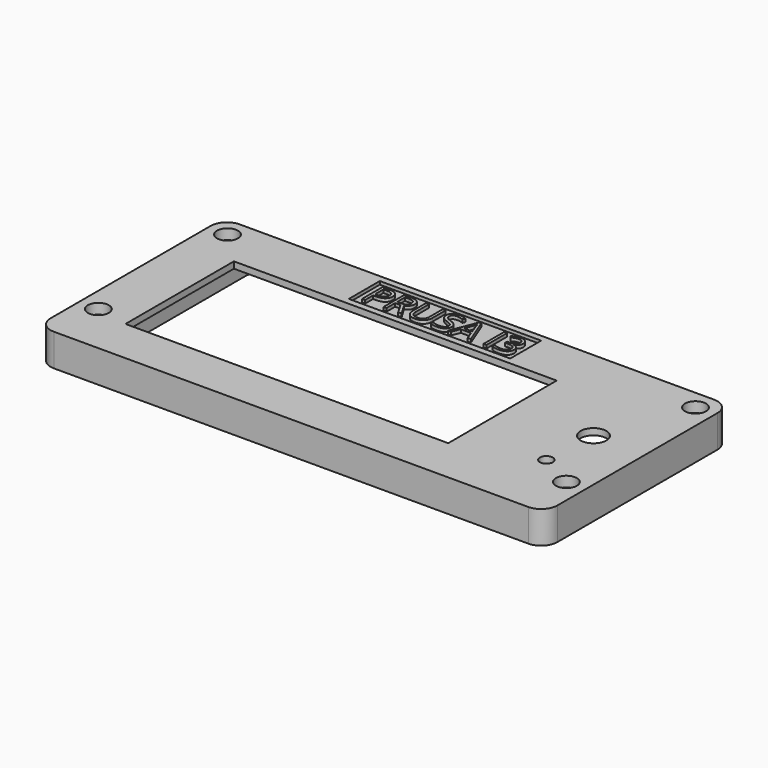
from build123d import *

# Parameters (mm, degrees)
F0_W           = 157
F0_H           = 72
F1_DEPTH       = 10
F2_W           = 100
F2_H           = 42
F2_R           = 4
F3_DEPTH       = 10.001
F4_R           = 4
F4_W           = 100
F4_H           = 42
F5_DEPTH       = 8
F6_R           = 5
F8_D           = 3.3
F8_DEPTH       = 12
F8_CBORE_D     = 6.5
F8_CBORE_DEPTH = 3.2
F8_TIP         = 0.9914200214
F9_W           = 50
F9_H           = 12
F10_DEPTH      = 1
F11_TEXT_SIZE  = 11.1111111111
F12_DEPTH      = 1
F13_R          = 2
F15_D          = 4


# Not quite as in the source:
# - Text() gives the source's letters only with a copy of the font that has no kerning and outlines rounded to 1/6400 em; it was checked with that copy


with BuildPart() as f1:
    # F0 (on Top) → F1 (new body)
    with BuildSketch(Plane.XY):
        with Locations((3.5, 8.5)):
            Rectangle(F0_W, F0_H)
    extrude(amount=F1_DEPTH)

    # F2 (on face) → F3 (cut, through all)
    with BuildSketch(Plane.XY.offset(10)):
        with Locations((-9, 7.5)):
            Rectangle(F2_W, F2_H)
        with Locations((66, 11.5)):
            Circle(F2_R)
    extrude(amount=-F3_DEPTH, mode=Mode.SUBTRACT)

    # F4 (on face) → F5 (cut)
    with BuildSketch(Plane(origin=(0, 0, 0), x_dir=(1, 0, 0), z_dir=(0, 0, -1))):
        with BuildLine():
            Line((71, 25.5), (-64, 25.5))
            Line((-64, 25.5), (-64, -41.5))
            Line((-64, -41.5), (70.8038475773, -41.5))
            ThreePointArc((70.8038475773, -41.5), (71.3859855926, -34.6645246646), (78, -32.8431457505))
            Line((78, -32.8431457505), (78, 5.5))
            Line((78, 5.5), (71, 5.5))
            Line((71, 5.5), (71, 25.5))
        make_face()
        with Locations((66, -11.5)):
            Circle(F4_R, mode=Mode.SUBTRACT)
        with Locations((-9, -7.5)):
            Rectangle(F4_W, F4_H, mode=Mode.SUBTRACT)
    extrude(amount=-F5_DEPTH, mode=Mode.SUBTRACT)

    # F6
    f6_edges = [f1.edges().sort_by_distance(p)[0] for p in [
        (-75, -27.5, 5),
        (-75, 44.5, 5),
        (82, 44.5, 5),
        (82, -27.5, 5),
    ]]
    fillet(f6_edges, radius=F6_R)

    # F8
    with Locations(Plane.XY.offset(10)):
        with Locations((-69, 38.5), (-69, -11.5), (76, 38.5), (76, -11.5)):
            CounterBoreHole(F8_D / 2, F8_CBORE_D / 2, F8_CBORE_DEPTH, depth=F8_DEPTH)
            with Locations((0, 0, -(F8_DEPTH + F8_TIP / 2))):  # 118° drill point
                Cone(0, F8_D / 2, F8_TIP, mode=Mode.SUBTRACT)

    # F9 (on face) → F10 (cut)
    with BuildSketch(Plane.XY.offset(10)):
        with Locations((0, 36.5)):
            Rectangle(F9_W, F9_H)
    extrude(amount=-F10_DEPTH, mode=Mode.SUBTRACT)

    # F11 (on face) → F12 (join, through all)
    with BuildSketch(Plane.XY.offset(9)):
        with Locations((-23.5911458333, 32.5)):
            Text('PRUSA I3', F11_TEXT_SIZE, font='Open Sans', text_align=(TextAlign.LEFT, TextAlign.BOTTOM))
    extrude(amount=F12_DEPTH)

    # F13
    f13_edges = [f1.edges().sort_by_distance(p)[0] for p in [
        (71, -5.5, 4),
        (78, -5.5, 4),
        (71, -25.5, 4),
        (78, 32.843146, 4),
        (70.803848, 41.5, 4),
        (-64, -25.5, 4),
        (-64, 41.5, 4),
    ]]
    fillet(f13_edges, radius=F13_R)

    # F15 (through all)
    with Locations(Plane.XY.offset(10)):
        with Locations((65, -5.5)):
            Hole(F15_D / 2)


solid = f1.part
